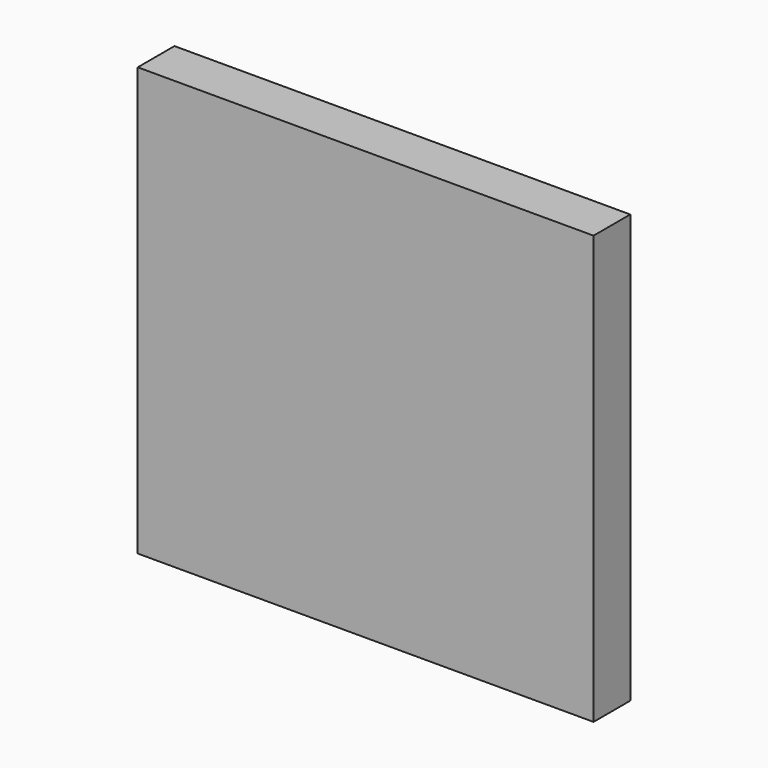
from build123d import *

# Parameters (mm, degrees)
F1_DEPTH = 2.54
F2_W     = 50.4335446749
F2_H     = 47.3673532251
F3_DEPTH = 5.08


# Not quite as in the source:
# - a feature names something its author has since deleted; it is built from what else it names


with BuildPart() as f1:
    # F0 (on Front) → F1 (new body)
    with BuildSketch(Plane.XZ):
        with BuildLine():
            Line((20.2425401959, 37.2512835941), (20.2425401959, 37.8724660293))
            ThreePointArc((20.2425401959, 37.8724660293), (25.0827531799, 5.42177238), (30.7611451277, 37.7363363557))
            Line((30.7611451277, 37.7363363557), (30.7611451277, 37.1095434926))
            ThreePointArc((30.7611451277, 37.1095434926), (25.0818490069, 6.0124710706), (20.2425401959, 37.2512835941))
        make_face()
    extrude(amount=F1_DEPTH)



with BuildPart() as f1b:
    # F0 (on Front) → F1, piece 2 (new body)
    with BuildSketch(Plane.XZ):
        with BuildLine():
            add(Edge.make_bspline(
                [(23.0514407158, 36.9153022766), (23.0000338532, 37.1051377654), (22.8899891699, 37.5115112571), (22.3511496369, 38.0986562322), (21.9858249437, 38.8447480675), (21.809539247, 39.6368045254), (21.813039047, 40.2648522584), (21.9686906382, 41.0721339012), (22.3787637159, 41.6567525791), (22.9775021785, 42.3782255437), (24.3228887053, 43.1166905037), (24.9982483073, 43.5418154349), (26.1666914194, 43.3968309792), (26.5298273051, 43.5335722369), (27.3608892448, 43.7811862144), (27.7584279708, 44.0883300962), (28.4498141772, 44.888079071), (28.5154236724, 45.4440168979), (28.92320837, 45.7942132009), (29.1466340423, 45.9860861301)],
                knots=[0, 0, 0, 0, 0.0514453921, 0.110127162, 0.171056953, 0.2301961795, 0.2830754093, 0.3422146359, 0.3975195588, 0.462072024, 0.5436046033, 0.6044006336, 0.6730540413, 0.7162652895, 0.7757385566, 0.8250838091, 0.8914195533, 0.940508657, 1, 1, 1, 1], degree=3))
            add(Edge.make_bspline(
                [(23.0514407158, 36.9153022766), (23.1528130098, 37.1260630271), (23.3607025921, 37.5582813649), (23.8028016121, 38.2012565529), (24.2676415464, 38.8465973471), (24.884509448, 39.3154758933), (25.8539932072, 39.587992103), (26.6019896914, 39.789301054), (27.3090151116, 39.8252756175), (27.3994263447, 39.9436529244), (27.6052961291, 40.0398924739), (27.6778788081, 40.2229303085), (27.9076828587, 40.3941993708), (28.0482787639, 40.498983115)],
                knots=[0, 0, 0, 0, 0.1035691547, 0.2123948021, 0.3213905308, 0.4288085843, 0.5510126252, 0.6639710224, 0.7625503685, 0.8077072913, 0.8630127537, 0.9161901374, 1, 1, 1, 1], degree=3))
            add(Edge.make_bspline(
                [(30.6448712945, 42.7375696599), (30.6857665771, 42.5799177306), (30.8089747033, 42.1049485515), (30.8481597012, 39.4706811929), (30.0006358069, 38.420435968), (29.0935620801, 37.4311516729), (27.7548428286, 36.4854500621), (27.5414798642, 37.1199299693), (28.1281216554, 38.0924200775), (28.2006198304, 39.4485309647), (28.0967658775, 40.1646452117), (28.0482787639, 40.498983115)],
                knots=[0, 0, 0, 0, 0.0811360963, 0.2444444876, 0.3629376576, 0.4864205288, 0.6058252757, 0.6665851424, 0.7746786569, 0.8948024484, 1, 1, 1, 1], degree=3))
            Line((30.6448712945, 42.7375696599), (28.9366003126, 41.7854189873))
            add(Edge.make_bspline(
                [(29.2866565287, 44.8379032314), (29.3276194284, 44.1605744561), (29.401104426, 42.9454870543), (29.0791063228, 42.1413182507), (28.9366003126, 41.7854189873)],
                knots=[0, 0, 0, 0, 0.5574321438, 1, 1, 1, 1], degree=3))
            Line((29.2866565287, 44.8379032314), (29.1466340423, 45.9860861301))
        make_face()
    extrude(amount=F1_DEPTH)


with BuildPart() as f1c:
    # F0 (on Front) → F1, piece 3 (new body)
    with BuildSketch(Plane.XZ):
        Polygon((33.2574028222, 26.435288895), (21.8032617122, 33.1698432565), (21.6212328523, 32.8617952764), (33.0605612282, 26.1021732809), align=None)
    extrude(amount=F1_DEPTH)


with BuildPart() as f1d:
    # F0 (on Front) → F1, piece 4 (new body)
    with BuildSketch(Plane.XZ):
        Polygon((33.228403627, 25.4895458259), (20.1059635729, 33.1698432565), (19.9089177924, 32.8258842821), (33.0227315426, 25.1305289567), align=None)
    extrude(amount=F1_DEPTH)


with BuildPart() as f1e:
    # F0 (on Front) → F1, piece 5 (new body)
    with BuildSketch(Plane.XZ):
        Polygon((33.2112317713, 24.5790107882), (18.4418894351, 33.1698432565), (18.2448436546, 32.8258842821), (32.9815978057, 24.1781665627), align=None)
    extrude(amount=F1_DEPTH)


with BuildPart() as f1f:
    # F0 (on Front) → F1, piece 6 (new body)
    with BuildSketch(Plane.XZ):
        Polygon((33.2125796453, 23.5776652022), (16.7505238205, 33.1698432565), (16.55347804, 32.8258842821), (33.0227315426, 23.2462703429), align=None)
    extrude(amount=F1_DEPTH)


with BuildPart() as f1g:
    # F0 (on Front) → F1, piece 7 (new body)
    with BuildSketch(Plane.XZ):
        Polygon((33.0227315426, 22.7067601114), (15.0789320469, 33.1698432565), (14.8818862664, 32.8258842821), (32.8367611378, 22.3821340801), align=None)
    extrude(amount=F1_DEPTH)


with BuildPart() as f1h:
    # F0 (on Front) → F1, piece 8 (new body)
    with BuildSketch(Plane.XZ):
        Polygon((33.3749822633, 17.101256154), (17.9576072842, 26.0595865548), (17.7897735171, 25.7666194572), (33.1791992282, 16.7595014014), align=None)
    extrude(amount=F1_DEPTH)


with BuildPart() as f1i:
    # F0 (on Front) → F1, piece 9 (new body)
    with BuildSketch(Plane.XZ):
        Polygon((33.3168466854, 16.1849598837), (17.9576072842, 25.1305289567), (17.76074414, 24.7868887884), (33.1290174507, 15.857089118), align=None)
    extrude(amount=F1_DEPTH)


with BuildPart() as f1j:
    # F0 (on Front) → F1, piece 10 (new body)
    with BuildSketch(Plane.XZ):
        Polygon((33.195942283, 15.2338305576), (17.9576072842, 24.1281539202), (17.7778732402, 23.8144139492), (33.0227315426, 14.9314775283), align=None)
    extrude(amount=F1_DEPTH)


with BuildPart() as f1k:
    # F0 (on Front) → F1, piece 11 (new body)
    with BuildSketch(Plane.XZ):
        Polygon((33.1469401717, 14.2789520323), (17.9576072842, 23.124800995), (17.7778732402, 22.811061024), (32.9511492616, 13.9945653465), align=None)
    extrude(amount=F1_DEPTH)


with BuildPart() as f1l:
    # F0 (on Front) → F1, piece 12 (new body)
    with BuildSketch(Plane.XZ):
        Polygon((33.0789424479, 13.332221657), (17.9576072842, 22.1720617265), (17.7778732402, 21.8583217555), (32.8649446067, 13.0281655517), align=None)
    extrude(amount=F1_DEPTH)


with BuildPart() as f1m:
    # F0 (on Front) → F1, piece 13 (new body)
    with BuildSketch(Plane.XZ):
        Polygon((29.7699026556, 10.0402957994), (17.841456458, 17.0968454331), (17.6537100383, 16.7688825837), (29.6143469321, 9.7685649275), align=None)
    extrude(amount=F1_DEPTH)


with BuildPart() as f1n:
    # F0 (on Front) → F1, piece 14 (new body)
    with BuildSketch(Plane.XZ):
        Polygon((28.8687120376, 9.5914553699), (17.841456458, 16.0501636565), (17.62953414, 15.6799693944), (28.7197476416, 9.3312384888), align=None)
    extrude(amount=F1_DEPTH)


with BuildPart() as f1o:
    # F0 (on Front) → F1, piece 15 (new body)
    with BuildSketch(Plane.XZ):
        Polygon((28.0626742242, 9.0640343876), (17.841456458, 15.0034837425), (17.6629371227, 14.6916391278), (27.9221774879, 8.8186091482), align=None)
    extrude(amount=F1_DEPTH)


with BuildPart() as f1p:
    # F0 (on Front) → F1, piece 16 (new body)
    with BuildSketch(Plane.XZ):
        Polygon((27.2564003965, 8.6249213116), (17.841456458, 14.0502564609), (17.6134166067, 13.6519074561), (27.0437242973, 8.2534103148), align=None)
    extrude(amount=F1_DEPTH)


with BuildPart() as f1q:
    # F0 (on Front) → F1, piece 17 (new body)
    with BuildSketch(Plane.XZ):
        Polygon((26.3865872887, 8.0787168843), (17.974415794, 13.0163198337), (17.7836155065, 12.6830223674), (26.1909458786, 7.7369627543), align=None)
    extrude(amount=F1_DEPTH)


with BuildPart() as f1r:
    # F0 (on Front) → F1, piece 18 (new body)
    with BuildSketch(Plane.XZ):
        Polygon((25.4722088575, 7.5785773806), (17.8834367543, 12.0687354356), (17.6850601811, 11.7222034147), (25.2775834555, 7.3757688617), align=None)
    extrude(amount=F1_DEPTH)


with BuildPart() as f1s:
    # F0 (on Front) → F1, piece 19 (new body)
    with BuildSketch(Plane.XZ):
        Polygon((33.1177413464, 12.4160759151), (17.9576072842, 21.0946835577), (17.7778732402, 20.7905191013), (20.1059635729, 19.4568124362), (17.7778732402, 17.5819434226), (30.4401450117, 10.1709731341), (33.1177413464, 12.0856873691), align=None)
        Polygon((22.9995213449, 15.0064639747), (23.3056563884, 17.5909493119), (28.043365106, 14.8232029751), (27.7810785919, 12.1866026893), align=None, mode=Mode.SUBTRACT)
    extrude(amount=F1_DEPTH)


with BuildPart() as f1t:
    # F0 (on Front) → F1, piece 20 (new body)
    with BuildSketch(Plane.XZ):
        Polygon((33.0227315426, 21.6672029346), (14.4121274352, 32.5775519013), (14.2134002971, 32.2306579844), (19.9089177924, 28.9678337124), (17.6128353924, 26.8874038011), (33.2432746912, 17.7152600915), (33.4723107517, 18.047504127), (30.8126039797, 19.594566601), align=None)
        Polygon((23.1198072433, 24.0452848375), (23.1421533972, 26.9667506218), (28.0626975, 24.0813326091), (27.9988050461, 21.2257355452), align=None, mode=Mode.SUBTRACT)
    extrude(amount=F1_DEPTH)


with BuildPart() as f1u:
    # F0 (on Front) → F1, piece 21 (new body)
    with BuildSketch(Plane.XZ):
        Polygon((23.0246130377, 33.5312858224), (23.0454113334, 33.2837961614), (23.0454113334, 32.939273864), (33.1866306884, 27.1296144809), (33.3058785922, 27.3377711162), (31.3267968595, 28.6425240338), (36.3370403647, 31.5886884928), (36.3370403647, 33.0705903471), (28.0454419553, 33.0705903471), (28.0454419553, 34.5877744257), (23.0461130826, 34.737955403), align=None)
        Polygon((23.2625063509, 33.2837961614), (23.2625063509, 33.5312858224), (23.2625063509, 34.509293735), (27.8020184487, 34.3729257584), (27.8020184487, 30.6832194328), align=None, mode=Mode.SUBTRACT)
    extrude(amount=F1_DEPTH)


with BuildPart() as f1_1:
    add(f1.part)

    add(f1b.part)  # F3 merges F1b

    add(f1c.part)  # F3 merges F1c

    add(f1d.part)  # F3 merges F1d

    add(f1e.part)  # F3 merges F1e

    add(f1f.part)  # F3 merges F1f

    add(f1g.part)  # F3 merges F1g

    add(f1h.part)  # F3 merges F1h

    add(f1i.part)  # F3 merges F1i

    add(f1j.part)  # F3 merges F1j

    add(f1k.part)  # F3 merges F1k

    add(f1l.part)  # F3 merges F1l

    add(f1m.part)  # F3 merges F1m

    add(f1n.part)  # F3 merges F1n

    add(f1o.part)  # F3 merges F1o

    add(f1p.part)  # F3 merges F1p

    add(f1q.part)  # F3 merges F1q

    add(f1r.part)  # F3 merges F1r

    add(f1s.part)  # F3 merges F1s

    add(f1t.part)  # F3 merges F1t

    add(f1u.part)  # F3 merges F1u
    # F2 (on face) → F3 (join)
    with BuildSketch(Plane.XZ.offset(2.54)):
        with Locations((27.7318180306, 26.7485658405)):
            Rectangle(F2_W, F2_H)
    extrude(amount=F3_DEPTH)


solid = f1_1.part
